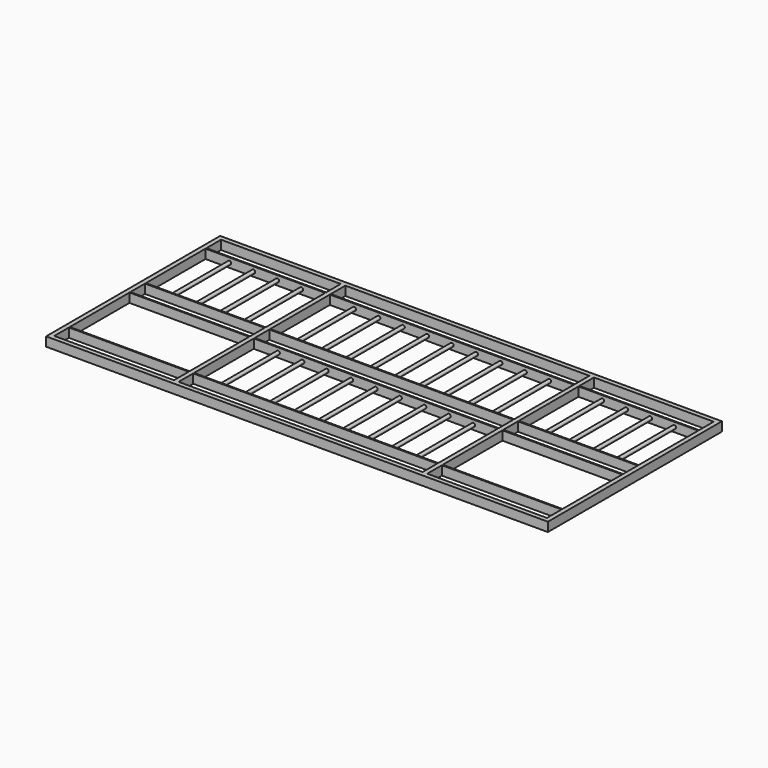
from build123d import *

# Parameters (mm, degrees)
F0_W     = 655
F0_H     = 6
F0_W_2   = 25
F1_DEPTH = 50
F4_R     = 9.525
F5_DEPTH = 408
F6_R     = 9.525
F7_DEPTH = 408
F8_R     = 9.525
F9_DEPTH = 408


# Not quite as in the source:
# - a feature names something its author has since deleted; it is built from what else it names
# - the program builds the solid bodies; features that only make, move or delete a surface that nothing else refers to are left out


with BuildPart() as f1:
    # F0 (on Top) → F1 (new body)
    with BuildSketch(Plane.XY):
        Polygon((0, 1190), (0, 0), (680, 0), (705, 0), (705, 25), (705, 125), (705, 131), (705, 539), (705, 545), (705, 645), (705, 651), (705, 1059), (705, 1065), (705, 1165), (705, 1190), (680, 1190), align=None)
        Polygon((25, 1065), (25, 1165), (680, 1165), (680, 1065), (680, 1059), (680, 651), (680, 645), (680, 545), (680, 539), (680, 131), (680, 125), (680, 25), (25, 25), (25, 125), (25, 131), (25, 539), (25, 545), (25, 645), (25, 651), (25, 1059), align=None, mode=Mode.SUBTRACT)
        Polygon((705, 25), (705, 0), (1360, 0), (1385, 0), (2040, 0), (2065, 0), (2065, 25), (2065, 125), (2065, 131), (2065, 539), (2065, 545), (2065, 645), (2065, 651), (2065, 1059), (2065, 1065), (2065, 1165), (2065, 1190), (2040, 1190), (1385, 1190), (1360, 1190), (705, 1190), (705, 1165), (1360, 1165), (1385, 1165), (2040, 1165), (2040, 1065), (2040, 1059), (2040, 651), (2040, 645), (2040, 545), (2040, 539), (2040, 131), (2040, 125), (2040, 25), (1385, 25), (1360, 25), align=None)
        Polygon((2065, 25), (2065, 0), (2745, 0), (2745, 1190), (2065, 1190), (2065, 1165), (2720, 1165), (2720, 1065), (2720, 1059), (2720, 651), (2720, 645), (2720, 545), (2720, 539), (2720, 131), (2720, 125), (2720, 25), align=None)
        with Locations((352.5, 542)):
            Rectangle(F0_W, F0_H)
        with Locations((352.5, 128)):
            Rectangle(F0_W, F0_H)
        with Locations((352.5, 648)):
            Rectangle(F0_W, F0_H)
        with Locations((352.5, 1062)):
            Rectangle(F0_W, F0_H)
        with Locations((1032.5, 648)):
            Rectangle(F0_W, F0_H)
        with Locations((1712.5, 648)):
            Rectangle(F0_W, F0_H)
        with Locations((1712.5, 542)):
            Rectangle(F0_W, F0_H)
        with Locations((1032.5, 542)):
            Rectangle(F0_W, F0_H)
        with Locations((2392.5, 542)):
            Rectangle(F0_W, F0_H)
        with Locations((2392.5, 648)):
            Rectangle(F0_W, F0_H)
        with Locations((2392.5, 1062)):
            Rectangle(F0_W, F0_H)
        with Locations((1712.5, 1062)):
            Rectangle(F0_W, F0_H)
        with Locations((1032.5, 1062)):
            Rectangle(F0_W, F0_H)
        with Locations((2392.5, 128)):
            Rectangle(F0_W, F0_H)
        with Locations((1032.5, 128)):
            Rectangle(F0_W, F0_H)
        with Locations((1712.5, 128)):
            Rectangle(F0_W, F0_H)
        with Locations((1372.5, 128)):
            Rectangle(F0_W_2, F0_H)
        with Locations((1372.5, 542)):
            Rectangle(F0_W_2, F0_H)
        with Locations((1372.5, 1062)):
            Rectangle(F0_W_2, F0_H)
        with Locations((1372.5, 648)):
            Rectangle(F0_W_2, F0_H)
    extrude(amount=F1_DEPTH)

    # F4 (on face) → F5 (join, through all)
    with BuildSketch(Plane(origin=(0, 651, 0), x_dir=(-1, 0, 0), z_dir=(0, 1, 0))):
        with Locations((-156, 25)):
            Circle(F4_R)
        with Locations((-287, 25)):
            Circle(F4_R)
        with Locations((-418, 25)):
            Circle(F4_R)
        with Locations((-549, 25)):
            Circle(F4_R)
        with Locations((-2196, 25)):
            Circle(F4_R)
        with Locations((-2327, 25)):
            Circle(F4_R)
        with Locations((-2458, 25)):
            Circle(F4_R)
        with Locations((-2589, 25)):
            Circle(F4_R)
    extrude(amount=F5_DEPTH)

    # F6 (on face) → F7 (join, through all)
    with BuildSketch(Plane(origin=(0, 131, 0), x_dir=(-1, 0, 0), z_dir=(0, 1, 0))):
        with Locations((-838.5, 25)):
            Circle(F6_R)
        with Locations((-972, 25)):
            Circle(F6_R)
        with Locations((-1105.5, 25)):
            Circle(F6_R)
        with Locations((-1239, 25)):
            Circle(F6_R)
        with Locations((-1372.5, 25)):
            Circle(F6_R)
        with Locations((-1506, 25)):
            Circle(F6_R)
        with Locations((-1639.5, 25)):
            Circle(F6_R)
        with Locations((-1773, 25)):
            Circle(F6_R)
        with Locations((-1906.5, 25)):
            Circle(F6_R)
    extrude(amount=F7_DEPTH)

    # F8 (on face) → F9 (join, through all)
    with BuildSketch(Plane(origin=(0, 651, 0), x_dir=(-1, 0, 0), z_dir=(0, 1, 0))):
        with Locations((-838.5, 25)):
            Circle(F8_R)
        with Locations((-972, 25)):
            Circle(F8_R)
        with Locations((-1105.5, 25)):
            Circle(F8_R)
        with Locations((-1239, 25)):
            Circle(F8_R)
        with Locations((-1372.5, 25)):
            Circle(F8_R)
        with Locations((-1506, 25)):
            Circle(F8_R)
        with Locations((-1639.5, 25)):
            Circle(F8_R)
        with Locations((-1773, 25)):
            Circle(F8_R)
        with Locations((-1906.5, 25)):
            Circle(F8_R)
    extrude(amount=F9_DEPTH)


solid = f1.part
